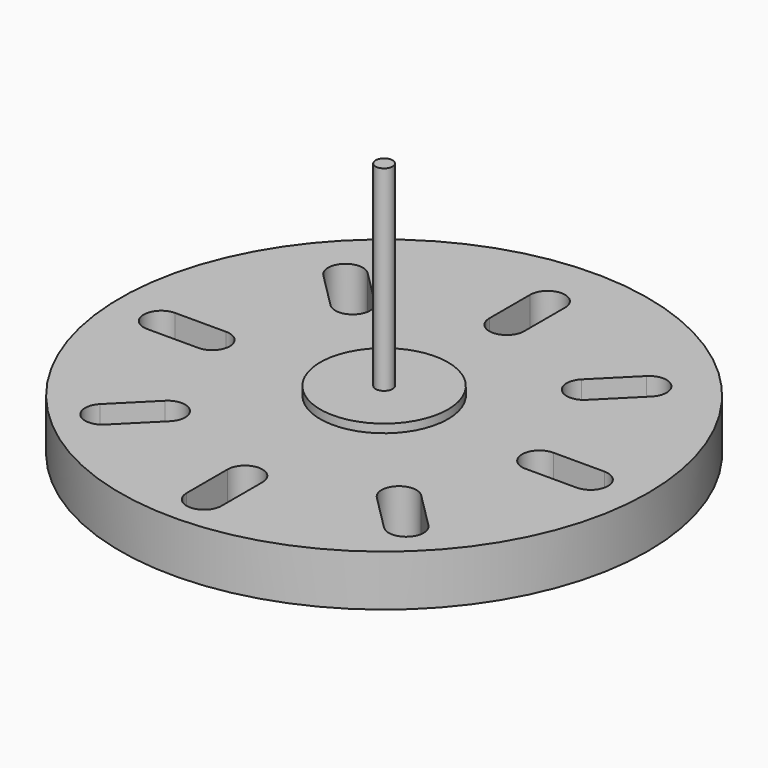
from build123d import *

# Parameters (mm, degrees)
F0_R     = 98.425
F0_R_2   = 20.6375
F1_DEPTH = 19.05
F2_R     = 20.6375
F3_DEPTH = 19.05
F4_R     = 3.175
F5_DEPTH = 76.2
F2_R_2   = 23.8125
F6_DEPTH = 3.175


with BuildPart() as f1:
    # F0 (on Top) → F1 (new body)
    with BuildSketch(Plane.XY):
        Circle(F0_R)
        with BuildLine():
            Line((-61.1991593756, -55.8554524149), (-47.728775194, -42.3850682333))
            ThreePointArc((-47.728775194, -42.3850682333), (-38.5363870385, -42.3850682333), (-38.5363870385, -51.5774563887))
            Line((-38.5363870385, -51.5774563887), (-52.0067712201, -65.0478405703))
            ThreePointArc((-52.0067712201, -65.0478405703), (-61.1991593756, -65.0478405703), (-61.1991593756, -55.8554524149))
        make_face(mode=Mode.SUBTRACT)
        with BuildLine():
            Line((-80.0486811947, 2.6513188053), (-60.9986811947, 2.6513188053))
            ThreePointArc((-60.9986811947, 2.6513188053), (-54.4986811947, -3.8486811947), (-60.9986811947, -10.3486811947))
            Line((-60.9986811947, -10.3486811947), (-80.0486811947, -10.3486811947))
            ThreePointArc((-80.0486811947, -10.3486811947), (-86.5486811947, -3.8486811947), (-80.0486811947, 2.6513188053))
        make_face(mode=Mode.SUBTRACT)
        with BuildLine():
            Line((-6.5, -83.8973623895), (-6.5, -64.8473623895))
            ThreePointArc((-6.5, -64.8473623895), (0, -58.3473623895), (6.5, -64.8473623895))
            Line((6.5, -64.8473623895), (6.5, -83.8973623895))
            ThreePointArc((6.5, -83.8973623895), (0, -90.3973623895), (-6.5, -83.8973623895))
        make_face(mode=Mode.SUBTRACT)
        with BuildLine():
            Line((52.0067712201, -65.0478405703), (38.5363870385, -51.5774563887))
            ThreePointArc((38.5363870385, -51.5774563887), (38.5363870385, -42.3850682333), (47.728775194, -42.3850682333))
            Line((47.728775194, -42.3850682333), (61.1991593756, -55.8554524149))
            ThreePointArc((61.1991593756, -55.8554524149), (61.1991593756, -65.0478405703), (52.0067712201, -65.0478405703))
        make_face(mode=Mode.SUBTRACT)
        with BuildLine():
            Line((80.0486811947, -10.3486811947), (60.9986811947, -10.3486811947))
            ThreePointArc((60.9986811947, -10.3486811947), (54.4986811947, -3.8486811947), (60.9986811947, 2.6513188053))
            Line((60.9986811947, 2.6513188053), (80.0486811947, 2.6513188053))
            ThreePointArc((80.0486811947, 2.6513188053), (86.5486811947, -3.8486811947), (80.0486811947, -10.3486811947))
        make_face(mode=Mode.SUBTRACT)
        with BuildLine():
            Line((-52.0067712201, 57.3504781808), (-38.5363870385, 43.8800939992))
            ThreePointArc((-38.5363870385, 43.8800939992), (-38.5363870385, 34.6877058438), (-47.728775194, 34.6877058438))
            Line((-47.728775194, 34.6877058438), (-61.1991593756, 48.1580900254))
            ThreePointArc((-61.1991593756, 48.1580900254), (-61.1991593756, 57.3504781808), (-52.0067712201, 57.3504781808))
        make_face(mode=Mode.SUBTRACT)
        Circle(F0_R_2, mode=Mode.SUBTRACT)
        with BuildLine():
            Line((61.1991593756, 48.1580900254), (47.728775194, 34.6877058438))
            ThreePointArc((47.728775194, 34.6877058438), (38.5363870385, 34.6877058438), (38.5363870385, 43.8800939992))
            Line((38.5363870385, 43.8800939992), (52.0067712201, 57.3504781808))
            ThreePointArc((52.0067712201, 57.3504781808), (61.1991593756, 57.3504781808), (61.1991593756, 48.1580900254))
        make_face(mode=Mode.SUBTRACT)
        with BuildLine():
            Line((6.5, 76.2), (6.5, 57.15))
            ThreePointArc((6.5, 57.15), (0, 50.65), (-6.5, 57.15))
            Line((-6.5, 57.15), (-6.5, 76.2))
            ThreePointArc((-6.5, 76.2), (0, 82.7), (6.5, 76.2))
        make_face(mode=Mode.SUBTRACT)
    extrude(amount=F1_DEPTH)


with BuildPart() as f3:
    # F2 (on face) → F3 (new body, through all)
    with BuildSketch(Plane.XY.offset(19.05)):
        Circle(F2_R)
    extrude(amount=-F3_DEPTH)

    # F4 (on face) → F5 (join)
    with BuildSketch(Plane.XY.offset(19.05)):
        Circle(F4_R)
    extrude(amount=F5_DEPTH)

    # F2 (on face) → F6 (join)
    with BuildSketch(Plane.XY.offset(19.05)):
        Circle(F2_R_2)
        Circle(F2_R, mode=Mode.SUBTRACT)
        Circle(F2_R)
    extrude(amount=F6_DEPTH)


solid = Compound([f1.part, f3.part])
